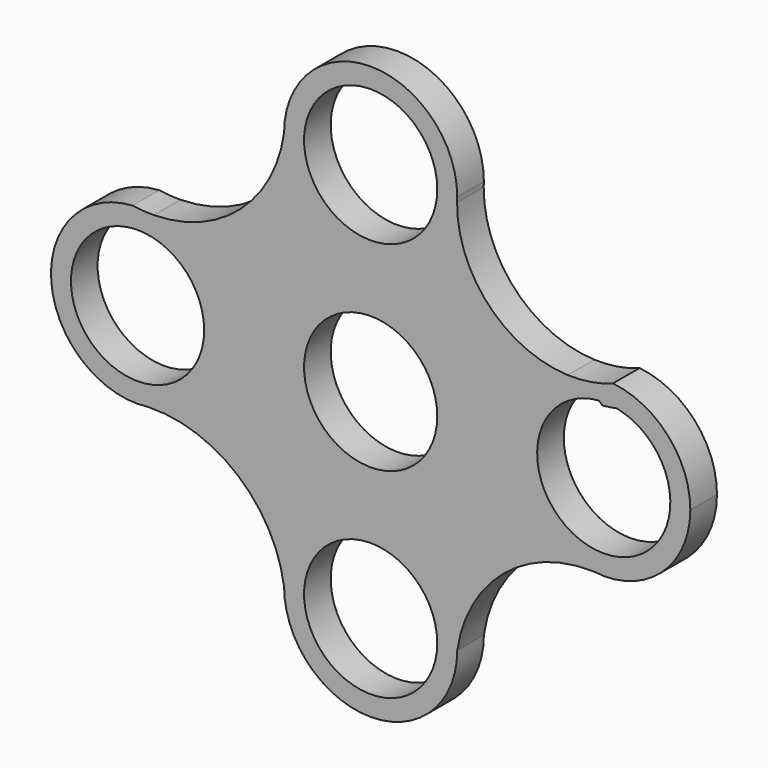
from build123d import *

# Parameters (mm, degrees)
F0_R     = 12.7
F1_DEPTH = 6.35


# Not quite as in the source:
# - a feature names something its author has since deleted; it is built from what else it names


with BuildPart() as f1:
    # F0 (on Front) → F1 (new body)
    with BuildSketch(Plane.XZ):
        with BuildLine():
            ThreePointArc((16.4814082308, 37.1287725662), (16.4903338535, 37.6145443772), (16.51, 38.1))
            ThreePointArc((16.51, 38.1), (0, 54.61), (-16.51, 38.1))
            ThreePointArc((-16.51, 38.1), (-0.4858240981, 21.5971494903), (16.4814082308, 37.1287725662))
        make_face()
        with Locations((0, 38.1)):
            Circle(F0_R, mode=Mode.SUBTRACT)
        with BuildLine():
            ThreePointArc((16.4814082308, 37.1287725662), (-0.4858240981, 21.5971494903), (-16.51, 38.1))
            ThreePointArc((-16.51, 38.1), (-24.8582581267, 22.5634685942), (-41.3111088486, 16.2088698662))
            ThreePointArc((-41.3111088486, 16.2088698662), (-31.7141609442, 10.5061174344), (-27.94, 0))
            ThreePointArc((-27.94, 0), (-32.0196049569, -10.8657893902), (-42.2422869864, -16.3617267808))
            ThreePointArc((-42.2422869864, -16.3617267808), (-25.2542323654, -22.3516257894), (-16.51, -38.1))
            ThreePointArc((-16.51, -38.1), (0, -21.59), (16.51, -38.1))
            ThreePointArc((16.51, -38.1), (25.2542323654, -22.3516257894), (42.2422869864, -16.3617267808))
            ThreePointArc((42.2422869864, -16.3617267808), (28.118646251, -2.4221859395), (37.5884063644, 15.0166118942))
            ThreePointArc((37.5884063644, 15.0166118942), (22.5582227264, 21.7995063444), (16.4814082308, 37.1287725662))
        make_face()
        Circle(F0_R, mode=Mode.SUBTRACT)
        with BuildLine():
            ThreePointArc((-27.94, 0), (-31.7141609442, 10.5061174344), (-41.3111088486, 16.2088698662))
            ThreePointArc((-41.3111088486, 16.2088698662), (-43.3621139683, 16.2630178255), (-45.4020575599, 16.4825266996))
            ThreePointArc((-45.4020575599, 16.4825266996), (-60.9531302457, -0.4762269364), (-44.45, -16.51))
            ThreePointArc((-44.45, -16.51), (-43.3477588373, -16.4118117369), (-42.2422869864, -16.3617267808))
            ThreePointArc((-42.2422869864, -16.3617267808), (-32.0196049569, -10.8657893902), (-27.94, 0))
        make_face()
        with Locations((-44.45, 0)):
            Circle(F0_R, mode=Mode.SUBTRACT)
        with BuildLine():
            ThreePointArc((46.209319854, 16.4159950552), (41.9691064238, 15.2835688562), (37.5884063644, 15.0166118942))
            ThreePointArc((37.5884063644, 15.0166118942), (28.118646251, -2.4221859395), (42.2422869864, -16.3617267808))
            ThreePointArc((42.2422869864, -16.3617267808), (43.3477588373, -16.4118117369), (44.45, -16.51))
            ThreePointArc((44.45, -16.51), (56.1243329574, -11.6743329574), (60.96, 0))
            ThreePointArc((60.96, 0), (56.7306040322, 11.0348024271), (46.209319854, 16.4159950552))
        make_face()
        with BuildLine():
            ThreePointArc((46.9166774243, 12.4581500426), (43.685710075, -12.6769815378), (43.4979424401, 12.6642641477))
            ThreePointArc((43.4979424401, 12.6642641477), (43.8445127875, 12.3613055932), (44.1938141149, 12.0614998657))
            ThreePointArc((44.1938141149, 12.0614998657), (45.5606208941, 12.2229266237), (46.9166774243, 12.4581500426))
        make_face(mode=Mode.SUBTRACT)
        with BuildLine():
            ThreePointArc((-16.51, -38.1), (0, -54.61), (16.51, -38.1))
            ThreePointArc((16.51, -38.1), (0, -21.59), (-16.51, -38.1))
        make_face()
        with Locations((0, -38.1)):
            Circle(F0_R, mode=Mode.SUBTRACT)
    extrude(amount=F1_DEPTH)


solid = f1.part
